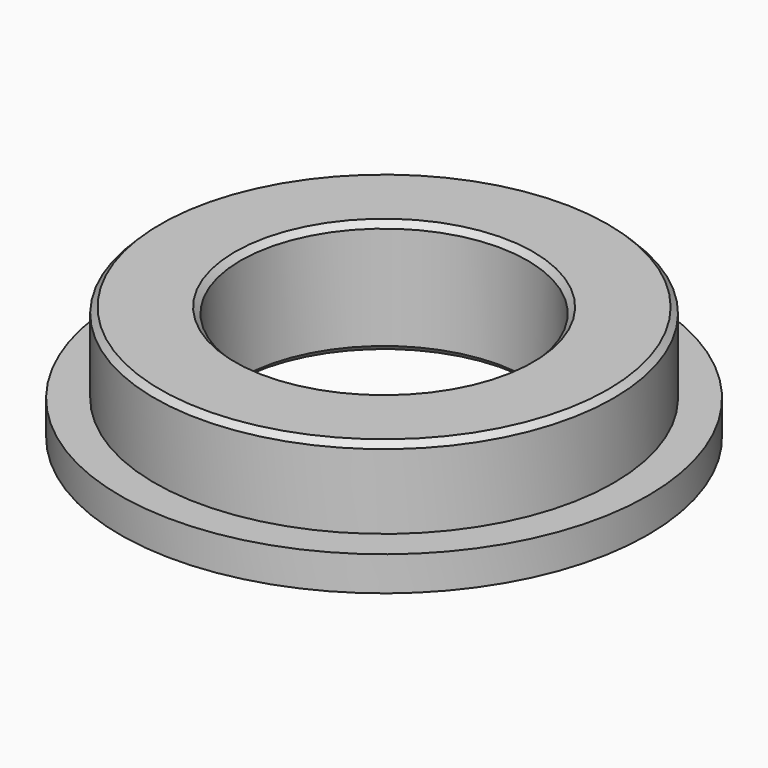
from build123d import *

# Parameters (mm, degrees)
F0_R     = 4
F1_DEPTH = 2
F0_R_2   = 4.6
F2_DEPTH = 0.6
F3_D     = 5
F4_SIZE  = 0.1


with BuildPart() as f1:
    # F0 (on Top) → F1 (new body)
    with BuildSketch(Plane.XY):
        Circle(F0_R)
    extrude(amount=F1_DEPTH)

    # F0 (on Top) → F2 (join)
    with BuildSketch(Plane.XY):
        Circle(F0_R_2)
        Circle(F0_R, mode=Mode.SUBTRACT)
    extrude(amount=F2_DEPTH)

    # F3 (through all)
    with Locations(Plane(origin=(0, 0, 0), x_dir=(1, 0, 0), z_dir=(0, 0, -1))):
        with Locations((0, 0)):
            Hole(F3_D / 2)

    # F4
    f4_edges = [f1.edges().sort_by_distance(p)[0] for p in [
        (-4, 0, 2),
        (-2.5, 0, 2),
        (-2.5, 0, 0),
    ]]
    chamfer(f4_edges, length=F4_SIZE)


solid = f1.part
